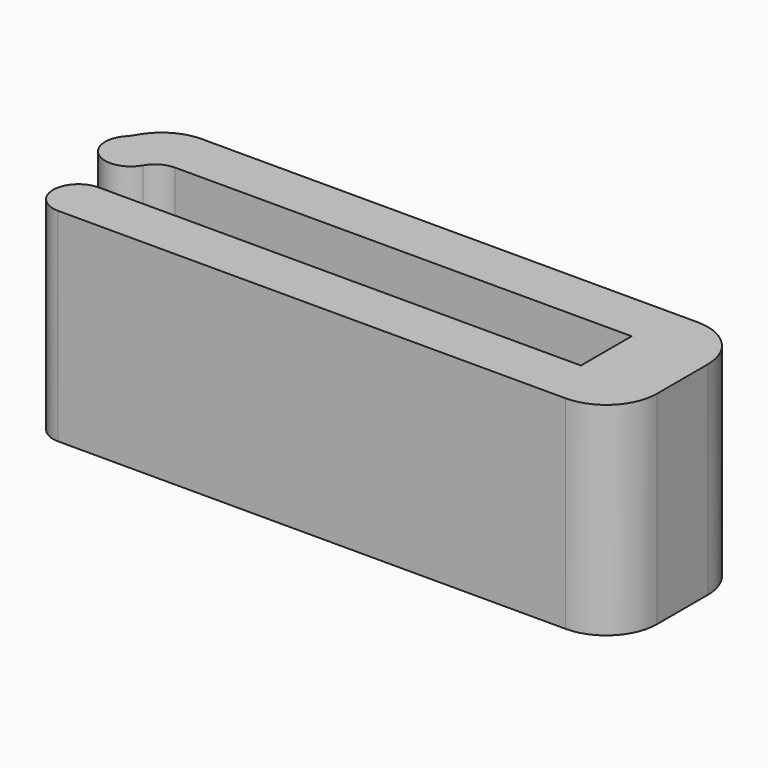
from build123d import *

# Parameters (mm, degrees)
F1_DEPTH = 8
F2_R     = 2
F3_R     = 1
F4_R     = 2
F5_R     = 0.99999


# Not quite as in the source:
# - a fillet or chamfer is up to 0.001 mm smaller than in the source, because OpenCascade refuses the exact size


with BuildPart() as f1:
    # F0 (on Top) → F1 (new body)
    with BuildSketch(Plane.XY):
        with BuildLine():
            Line((20, 0), (0, 0))
            Line((0, 0), (0, -2))
            Line((0, -2), (23, -2))
            Line((23, -2), (23, 4.5))
            Line((23, 4.5), (0, 4.5))
            Line((0, 4.5), (0, 3.478939205))
            ThreePointArc((0, 3.478939205), (-0.3538557851, 1.6956316782), (1.2766015908, 2.5))
            Line((1.2766015908, 2.5), (20, 2.5))
            Line((20, 2.5), (20, 0))
        make_face()
    extrude(amount=F1_DEPTH)

    # F2
    f2_edges = [f1.edges().sort_by_distance(p)[0] for p in [
        (23, -2, 4),
        (23, 4.5, 4),
        (0, 3.478939, 4),
    ]]
    fillet(f2_edges, radius=F2_R)

    # F3
    f3_edges = [f1.edges().sort_by_distance(p)[0] for p in [
        (1.276602, 2.5, 4),
    ]]
    fillet(f3_edges, radius=F3_R)

    # F4
    f4_edges = [f1.edges().sort_by_distance(p)[0] for p in [
        (0, 4.5, 4),
    ]]
    fillet(f4_edges, radius=F4_R)

    # F5 (radius 1 in the source; OpenCascade refuses exactly that, so slightly less here)
    f5_edges = [f1.edges().sort_by_distance(p)[0] for p in [
        (0, 0, 4),
        (0, -2, 4),
    ]]
    fillet(f5_edges, radius=F5_R)


solid = f1.part
